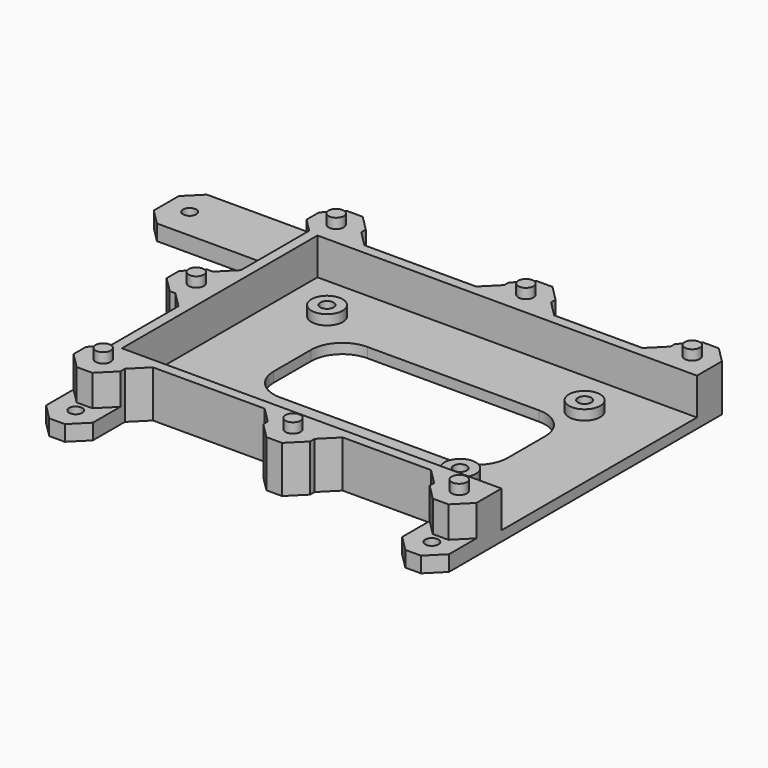
from build123d import *

# Parameters (mm, degrees)
F0_W          = 121.6
F0_H          = 78.3
F0_R          = 2.125
F1_DEPTH      = 3.2
F2_R          = 5
F2_R_2        = 2.125
F3_DEPTH      = 3.2
F5_DEPTH      = 4
F7_DEPTH      = 15
F8_R          = 2.425
F9_DEPTH      = 3.2
F10_T1_DEPTH  = 15
F10_T3_DEPTH  = 40.7168298797
F10_T8_DEPTH  = 40.7168298797
F10_T13_DEPTH = 40.7168298797
F11_W         = 15
F11_H         = 17.8
F11_R         = 2.125
F11_W_2       = 50
F11_H_2       = 20
F12_DEPTH     = 5
F13_SIZE      = 5


# Not quite as in the source:
# - a fillet or chamfer that OpenCascade refuses, or shapes differently, is made with other operations: its cross-section is extruded or revolved along the edge and cut away or added
# - a feature names something its author has since deleted; it is built from what else it names


with BuildPart() as f1:
    # F0 (on Top) → F1 (new body)
    with BuildSketch(Plane.XY):
        Rectangle(F0_W, F0_H)
        with Locations((35.5, -24.05)):
            Circle(F0_R, mode=Mode.SUBTRACT)
        with BuildLine():
            ThreePointArc((37.5, -7.5), (34.5710678119, -14.5710678119), (27.5, -17.5))
            Line((27.5, -17.5), (-27.5, -17.5))
            ThreePointArc((-27.5, -17.5), (-34.5710678119, -14.5710678119), (-37.5, -7.5))
            Line((-37.5, -7.5), (-37.5, 7.5))
            ThreePointArc((-37.5, 7.5), (-34.5710678119, 14.5710678119), (-27.5, 17.5))
            Line((-27.5, 17.5), (27.5, 17.5))
            ThreePointArc((27.5, 17.5), (34.5710678119, 14.5710678119), (37.5, 7.5))
            Line((37.5, 7.5), (37.5, -7.5))
        make_face(mode=Mode.SUBTRACT)
        with Locations((-45.72, 24.15)):
            Circle(F0_R, mode=Mode.SUBTRACT)
        with Locations((36.8, 24.15)):
            Circle(F0_R, mode=Mode.SUBTRACT)
    extrude(amount=F1_DEPTH)

    # F2 (on face) → F3 (join)
    with BuildSketch(Plane.XY.offset(3.2)):
        with Locations((-45.72, 24.15)):
            Circle(F2_R)
        with Locations((-45.72, 24.15)):
            Circle(F2_R_2, mode=Mode.SUBTRACT)
        with Locations((36.8, 24.15)):
            Circle(F2_R)
        with Locations((36.8, 24.15)):
            Circle(F2_R_2, mode=Mode.SUBTRACT)
        with Locations((35.5, -24.05)):
            Circle(F2_R)
        with Locations((35.5, -24.05)):
            Circle(F2_R_2, mode=Mode.SUBTRACT)
    extrude(amount=F3_DEPTH)

    # F4 (on face) → F5 (cut)
    with BuildSketch(Plane(origin=(0, 0, 0), x_dir=(1, 0, 0), z_dir=(0, 0, -1))):
        Polygon((-44.0312504626, -21.225), (-47.4087495374, -21.225), (-49.0974990748, -24.15), (-47.4087495374, -27.075), (-44.0312504626, -27.075), (-42.3425009252, -24.15), align=None)
        Polygon((38.4887495374, -21.225), (35.1112504626, -21.225), (33.4225009252, -24.15), (35.1112504626, -27.075), (38.4887495374, -27.075), (40.1774990748, -24.15), align=None)
        Polygon((33.8112504626, 21.125), (37.1887495374, 21.125), (38.8774990748, 24.05), (37.1887495374, 26.975), (33.8112504626, 26.975), (32.1225009252, 24.05), align=None)
    extrude(amount=-F5_DEPTH, mode=Mode.SUBTRACT)

    # F6 (on Top) → F7 (join)
    with BuildSketch(Plane.XY):
        Polygon((-60.8, 39.15), (60.8, 39.15), (60.8, 54.15), (45.8, 54.15), (45.8, 42.35), (7.5, 42.35), (7.5, 54.15), (-7.5, 54.15), (-7.5, 42.35), (-53.3, 42.35), (-53.3, 54.15), (-68.3, 54.15), (-68.3, 39.15), (-64, 39.15), (-64, 7.5), (-75.8, 7.5), (-75.8, -7.5), (-64, -7.5), (-64, -39.15), (-68.3, -39.15), (-68.3, -54.15), (-53.3, -54.15), (-53.3, -42.35), (-7.5, -42.35), (-7.5, -54.15), (7.5, -54.15), (7.5, -42.35), (45.8, -42.35), (45.8, -54.15), (60.8, -54.15), (60.8, -39.15), (-60.8, -39.15), align=None)
    extrude(amount=F7_DEPTH)

    # F8 (on face) → F9 (join)
    with BuildSketch(Plane.XY.offset(15)):
        with Locations((53.3, 46.65)):
            Circle(F8_R)
        with Locations((0, 46.65)):
            Circle(F8_R)
        with Locations((-60.8, 46.65)):
            Circle(F8_R)
        with Locations((-68.3, 0)):
            Circle(F8_R)
        with Locations((-60.8, -46.65)):
            Circle(F8_R)
        with Locations((0, -46.65)):
            Circle(F8_R)
        with Locations((53.3, -46.65)):
            Circle(F8_R)
    extrude(amount=F9_DEPTH)

    # F10: chamfer of 5 on 26 edges, made by hand

    # F10_s2 → F10_t1 (join)
    with BuildSketch(Plane.XY):
        Polygon((-12.5, -42.35), (-7.5, -47.35), (-7.5, -42.35), align=None)
        Polygon((7.5, -47.35), (12.5, -42.35), (7.5, -42.35), align=None)
        Polygon((40.8, -42.35), (45.8, -47.35), (45.8, -42.35), align=None)
        Polygon((-53.3, -47.35), (-48.3, -42.35), (-53.3, -42.35), align=None)
        Polygon((-69, -7.5), (-64, -12.5), (-64, -7.5), align=None)
        Polygon((-64, 12.5), (-69, 7.5), (-64, 7.5), align=None)
        Polygon((-48.3, 42.35), (-53.3, 47.35), (-53.3, 42.35), align=None)
        Polygon((-7.5, 47.35), (-12.5, 42.35), (-7.5, 42.35), align=None)
        Polygon((45.8, 47.35), (40.8, 42.35), (45.8, 42.35), align=None)
        Polygon((12.5, 42.35), (7.5, 47.35), (7.5, 42.35), align=None)
    extrude(amount=F10_T1_DEPTH)

    # F10_s4 → F10_t3 (cut)
    with BuildSketch(Plane.XY.offset(-12.8584149398)):
        Polygon((-75.8, -2.5), (-70.8, -7.5), (-75.8, -7.5), align=None)
        Polygon((-70.8, 7.5), (-75.8, 2.5), (-75.8, 7.5), align=None)
        Polygon((-63.3, 54.15), (-68.3, 49.15), (-68.3, 54.15), align=None)
        Polygon((-53.3, 49.15), (-58.3, 54.15), (-53.3, 54.15), align=None)
        Polygon((-2.5, 54.15), (-7.5, 49.15), (-7.5, 54.15), align=None)
        Polygon((7.5, 49.15), (2.5, 54.15), (7.5, 54.15), align=None)
        Polygon((50.8, 54.15), (45.8, 49.15), (45.8, 54.15), align=None)
        Polygon((60.8, 49.15), (55.8, 54.15), (60.8, 54.15), align=None)
        Polygon((60.8, -49.15), (55.8, -54.15), (60.8, -54.15), align=None)
        Polygon((50.8, -54.15), (45.8, -49.15), (45.8, -54.15), align=None)
        Polygon((2.5, -54.15), (7.5, -49.15), (7.5, -54.15), align=None)
        Polygon((-7.5, -49.15), (-2.5, -54.15), (-7.5, -54.15), align=None)
        Polygon((-58.3, -54.15), (-53.3, -49.15), (-53.3, -54.15), align=None)
        Polygon((-68.3, -49.15), (-63.3, -54.15), (-68.3, -54.15), align=None)
    extrude(amount=F10_T3_DEPTH, mode=Mode.SUBTRACT)


with BuildPart() as f10_tool6:
    # F10_s7 → F10_t8 (new body)
    with BuildSketch(Plane.XY.offset(-12.8584149398)):
        Polygon((-68.3, 44.15), (-63.3, 39.15), (-68.3, 39.15), align=None)
    extrude(amount=F10_T8_DEPTH)

    split(bisect_by=Plane.YZ.offset(-64), keep=Keep.BOTTOM)


with BuildPart() as f1_1:
    add(f1.part)

    # F10_t5: cut F10_tool6
    add(f10_tool6.part, mode=Mode.SUBTRACT)


with BuildPart() as f10_tool11:
    # F10_s12 → F10_t13 (new body)
    with BuildSketch(Plane.XY.offset(-12.8584149398)):
        Polygon((-63.3, -39.15), (-68.3, -44.15), (-68.3, -39.15), align=None)
    extrude(amount=F10_T13_DEPTH)

    split(bisect_by=Plane.YZ.offset(-64), keep=Keep.BOTTOM)


with BuildPart() as f1_2:
    add(f1_1.part)

    # F10_t10: cut F10_tool11
    add(f10_tool11.part, mode=Mode.SUBTRACT)

    # F11 (on Top) → F12 (join)
    with BuildSketch(Plane.XY):
        with Locations((53.3, -56.25)):
            Rectangle(F11_W, F11_H)
        with Locations((53.3, -57.65)):
            Circle(F11_R, mode=Mode.SUBTRACT)
        with Locations((-60.8, -56.25)):
            Rectangle(F11_W, F11_H)
        with Locations((-60.8, -57.65)):
            Circle(F11_R, mode=Mode.SUBTRACT)
        with Locations((-88.225, 44.15)):
            Rectangle(F11_W_2, F11_H_2)
        with Locations((-105.725, 44.15)):
            Circle(F11_R, mode=Mode.SUBTRACT)
    extrude(amount=F12_DEPTH)

    # F13
    f13_edges = [f1_2.edges().sort_by_distance(p)[0] for p in [
        (-68.3, -65.15, 2.5),
        (-53.3, -65.15, 2.5),
        (45.8, -65.15, 2.5),
        (60.8, -65.15, 2.5),
        (-113.225, 54.15, 2.5),
        (-113.225, 34.15, 2.5),
        (-64, 34.15, 2.5),
    ]]
    chamfer(f13_edges, length=F13_SIZE)


solid = f1_2.part
